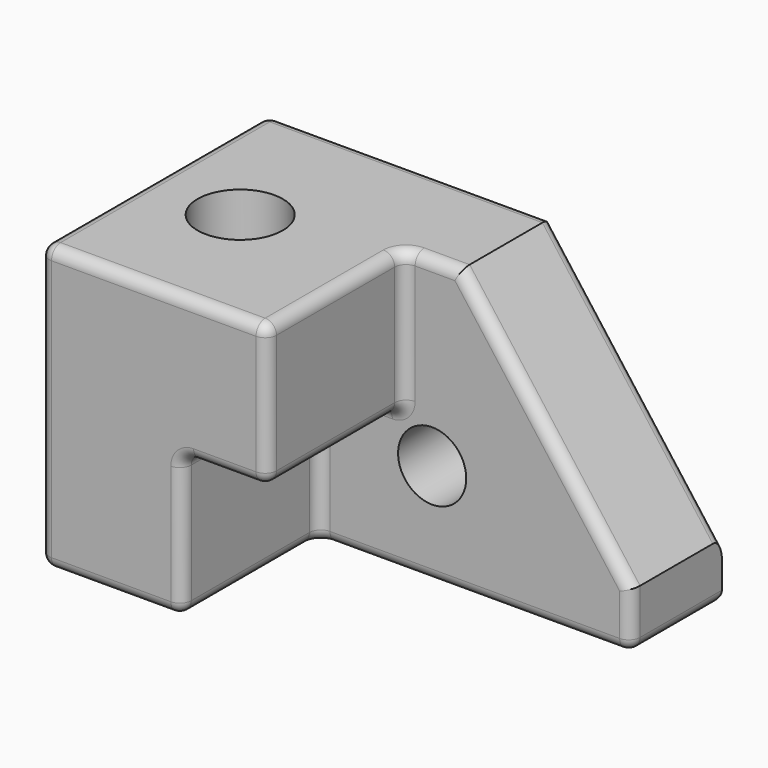
from build123d import *

# Parameters (mm, degrees)
F1_DEPTH = 127
F3_DEPTH = 76.2
F4_SIZE2 = 101.6
F4_SIZE  = 76.2
F5_R     = 5.08
F6_R     = 15.24
F7_DEPTH = 50.8
F8_R     = 19.05
F9_DEPTH = 127


with BuildPart() as f1:
    # F0 (on Front) → F1 (new body)
    with BuildSketch(Plane.XZ):
        Polygon((101.6, -63.5), (101.6, 63.5), (0, 63.5), (0, 0), (-38.1, 0), (-38.1, -63.5), align=None)
        Polygon((0, 0), (0, 63.5), (-101.6, 63.5), (-101.6, -63.5), (-38.1, -63.5), (-38.1, 0), align=None)
    extrude(amount=F1_DEPTH)

    # F2 (on face) → F3 (cut)
    with BuildSketch(Plane.XZ.offset(127)):
        Polygon((-38.1, 0), (-38.1, -63.5), (101.6, -63.5), (101.6, 63.5), (0, 63.5), (0, 0), align=None)
    extrude(amount=-F3_DEPTH, mode=Mode.SUBTRACT)

    # F4
    f4_edges = [f1.edges().sort_by_distance(p)[0] for p in [
        (101.6, -25.4, 63.5),
    ]]
    f4_side = f1.faces().sort_by_distance((-21.771429, -52.614286, 63.5))[0]
    chamfer(f4_edges, length=F4_SIZE, length2=F4_SIZE2, reference=f4_side)

    # F5
    f5_edges = [f1.edges().sort_by_distance(p)[0] for p in [
        (63.5, -50.8, 12.7),
        (63.5, 0, 12.7),
        (12.7, -50.8, 63.5),
        (0, -88.9, 63.5),
        (-50.8, -127, 63.5),
        (0, -127, 31.75),
        (0, -88.9, 0),
        (31.75, -50.8, -63.5),
        (101.6, -50.8, -50.8),
        (101.6, -25.4, -63.5),
        (-101.6, -127, 0),
        (-69.85, -127, -63.5),
        (-38.1, 0, 63.5),
        (-101.6, 0, 0),
        (0, 0, -63.5),
        (-101.6, -63.5, -63.5),
        (-38.1, -88.9, -63.5),
        (-101.6, -63.5, 63.5),
        (-38.1, -127, -31.75),
        (-19.05, -127, 0),
        (-38.1, -88.9, 0),
        (-19.05, -50.8, 0),
        (-38.1, -50.8, -31.75),
        (0, -50.8, 31.75),
    ]]
    fillet(f5_edges, radius=F5_R)

    # F6 (on face) → F7 (cut, through all)
    with BuildSketch(Plane.XZ.offset(50.8)):
        with Locations((12.7, -17.78)):
            Circle(F6_R)
    extrude(amount=-F7_DEPTH, mode=Mode.SUBTRACT)

    # F8 (on face) → F9 (cut, through all)
    with BuildSketch(Plane.XY.offset(63.5)):
        with Locations((-60.7483349741, -66.2939995527)):
            Circle(F8_R)
    extrude(amount=-F9_DEPTH, mode=Mode.SUBTRACT)


solid = f1.part
